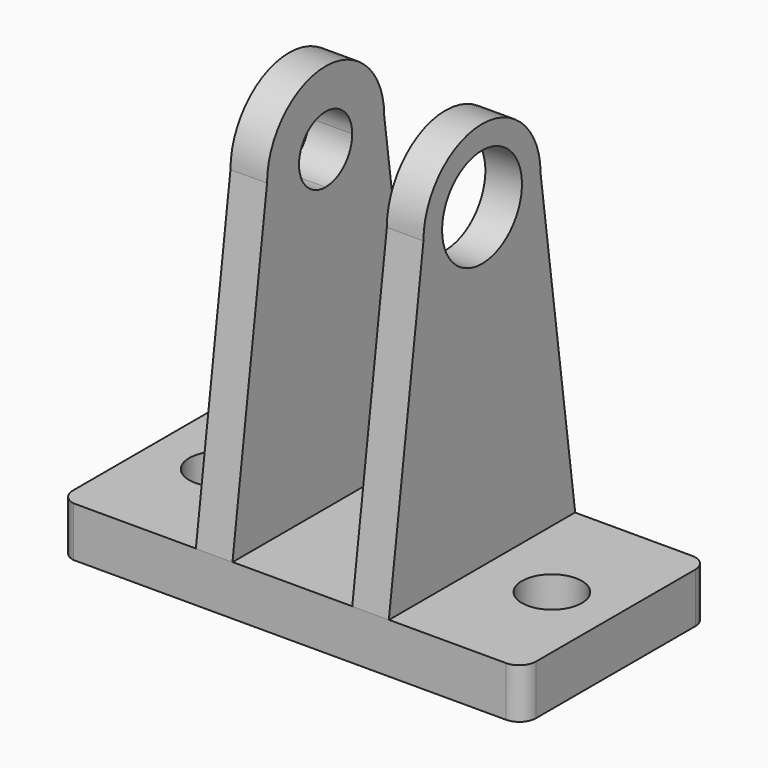
from build123d import *

# Parameters (mm, degrees)
F5_DEPTH = 15
F6_DEPTH = 11
F7_DEPTH = 11
F8_DEPTH = 13


# Not quite as in the source:
# - a feature of the source that left no trace in its solid (it failed there, or was rolled back) is left out


with BuildPart() as f5:
    # F0 (on Top) → F5 (new body)
    with BuildSketch(Plane.XY):
        with BuildLine():
            Line((-70, 30), (-70, 0))
            Line((-70, 0), (-70, -30))
            ThreePointArc((-70, -30), (-68.8225510753, -33.2230580629), (-65.8447586893, -34.9281216256))
            Line((-65.8447586893, -34.9281216256), (64.1552413107, -34.9281216256))
            ThreePointArc((64.1552413107, -34.9281216256), (67.6652703796, -33.4889776935), (69.154724634, -30))
            Line((69.154724634, -30), (69.154724634, 0))
            Line((69.154724634, 0), (69.154724634, 30))
            ThreePointArc((69.154724634, 30), (67.6652703796, 33.4889776935), (64.1552413107, 34.9281216256))
            Line((64.1552413107, 34.9281216256), (-65.8447586893, 34.9281216256))
            ThreePointArc((-65.8447586893, 34.9281216256), (-68.8225510753, 33.2230580629), (-70, 30))
        make_face()
        with BuildLine():
            ThreePointArc((-41, 0), (-50, -9), (-59, 0))
            ThreePointArc((-59, 0), (-50, 9), (-41, 0))
        make_face(mode=Mode.SUBTRACT)
        with BuildLine():
            ThreePointArc((59, 0), (50, -9), (41, 0))
            ThreePointArc((41, 0), (50, 9), (59, 0))
        make_face(mode=Mode.SUBTRACT)
    extrude(amount=-F5_DEPTH)

    # F2 (on offset) → F6 (join)
    with BuildSketch(Plane.YZ.offset(-18)):
        with BuildLine():
            Line((-35, 0), (0, 0))
            Line((0, 0), (35, 0))
            Line((35, 0), (22, 95))
            ThreePointArc((22, 95), (0, 117), (-22, 95))
            Line((-22, 95), (-35, 0))
        make_face()
        with BuildLine():
            ThreePointArc((15, 95), (10.6066017178, 84.3933982822), (0, 80))
            ThreePointArc((0, 80), (-10.6066017178, 84.3933982822), (-15, 95))
            ThreePointArc((-15, 95), (0, 110), (15, 95))
        make_face(mode=Mode.SUBTRACT)
    extrude(amount=-F6_DEPTH)

    # F4 (on offset) → F7 (join)
    with BuildSketch(Plane.YZ.offset(18)):
        with BuildLine():
            ThreePointArc((22, 95), (0, 117), (-22, 95))
            Line((-22, 95), (-35, 0))
            Line((-35, 0), (0, 0))
            Line((0, 0), (35, 0))
            Line((35, 0), (22, 95))
        make_face()
        with BuildLine():
            ThreePointArc((15, 95), (10.6066017178, 84.3933982822), (0, 80))
            ThreePointArc((0, 80), (-10.6066017178, 84.3933982822), (-15, 95))
            ThreePointArc((-15, 95), (0, 110), (15, 95))
        make_face(mode=Mode.SUBTRACT)
    extrude(amount=F7_DEPTH)

    # F2 (on offset) → F8 (join)
    with BuildSketch(Plane.YZ.offset(-18)):
        with BuildLine():
            ThreePointArc((-15, 95), (-10.6066017178, 84.3933982822), (0, 80))
            ThreePointArc((0, 80), (10.6066017178, 84.3933982822), (15, 95))
            ThreePointArc((15, 95), (0, 110), (-15, 95))
        make_face()
        with BuildLine():
            ThreePointArc((10, 95), (7.0710678119, 87.9289321881), (0, 85))
            ThreePointArc((0, 85), (-7.0710678119, 87.9289321881), (-10, 95))
            ThreePointArc((-10, 95), (0, 105), (10, 95))
        make_face(mode=Mode.SUBTRACT)
    extrude(amount=-F8_DEPTH)


solid = f5.part
